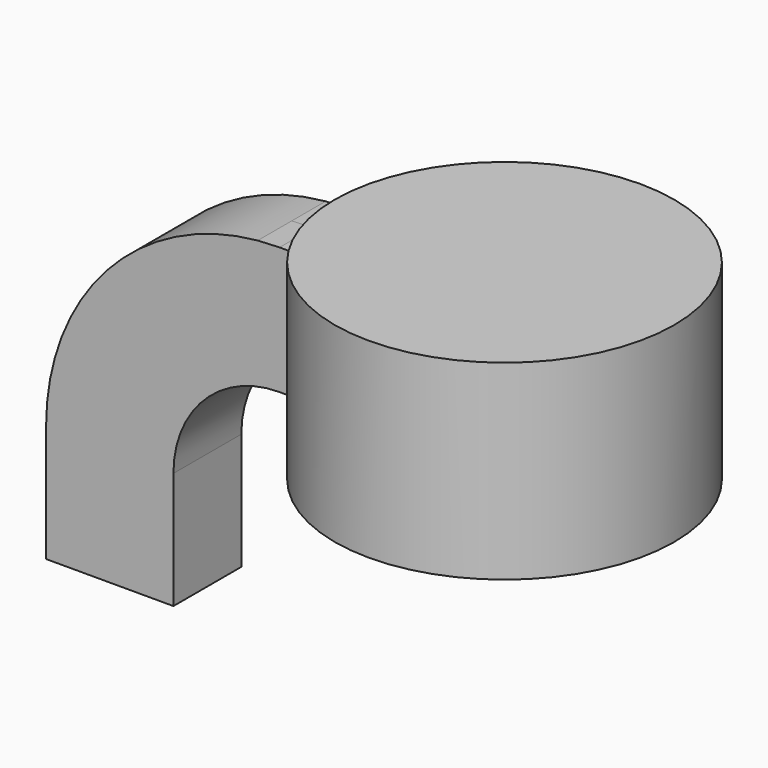
from build123d import *

# Parameters (mm, degrees)
F0_W     = 25.4
F0_H     = 19.05
F1_DEPTH = 6.35


# Not quite as in the source:
# - a feature of the source that left no trace in its solid (it failed there, or was rolled back) is left out


with BuildPart() as f1:
    # F0 (on Front) → F1 (new body, symmetric)
    with BuildSketch(Plane.XZ):
        with BuildLine():
            Line((22.225, 27.0002), (22.225, 9.525))
            Line((22.225, 9.525), (41.275, 9.525))
            Line((41.275, 9.525), (41.275, 27.0002))
            ThreePointArc((41.275, 27.0002), (45.9246798487, 38.2255201513), (57.15, 42.8752))
            Line((57.15, 42.8752), (60.325, 42.8752))
            Line((60.325, 42.8752), (60.325, 61.9252))
            Line((60.325, 61.9252), (57.15, 61.9252))
            add(Edge.make_bspline(
                [(53.8854342407, 61.7722898912), (54.9842067368, 61.8365871986), (56.0728453275, 61.8876096574), (57.15, 61.9252)],
                knots=[108.5245810491, 108.5245810491, 108.5245810491, 108.5245810491, 111.5045361635, 111.5045361635, 111.5045361635, 111.5045361635], degree=3))
            ThreePointArc((53.8854342407, 61.7722898912), (31.3258777096, 50.5133948686), (22.225, 27.0002))
        make_face()
        with Locations((73.025, 52.4002)):
            Rectangle(F0_W, F0_H)
    extrude(amount=F1_DEPTH, both=True)

    # F0 (on Front) → F2 (revolve)
    with BuildSketch(Plane.XZ):
        Polygon((85.725, 66.675), (85.725, 61.9252), (85.725, 42.8752), (85.725, 38.1), (111.125, 38.1), (111.125, 66.675), align=None)
    revolve(axis=Axis((85.725, 0, 52.3875), (0, 0, 1)))


solid = f1.part
